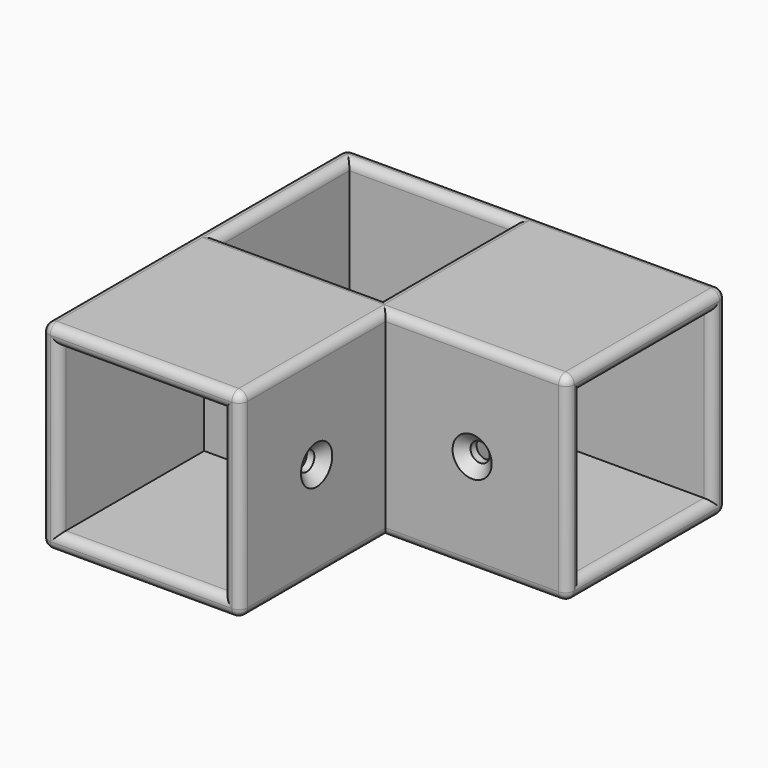
from build123d import *

# Parameters (mm, degrees)
F0_W                  = 34.2
F0_H                  = 34.2
F0_W_2                = 28.2
F0_H_2                = 28.2
F1_DEPTH              = 3
F2_DEPTH              = 31.2
F3_W                  = 34.2
F3_H                  = 34.2
F3_W_2                = 28.2
F3_H_2                = 28.2
F4_DEPTH              = 31.2
F5_W                  = 34.2
F5_H                  = 34.2
F5_W_2                = 28.2
F5_H_2                = 28.2
F6_DEPTH              = 31.2
F7_D                  = 3.3
F7_DEPTH              = 13.5
F7_CSINK_D            = 6.72
F7_CSINK_ANGLE        = 90
F7_TIP                = 0.9914200214
F7_ON_F5_D            = 3.3
F7_ON_F5_DEPTH        = 13.5
F7_ON_F5_CSINK_D      = 6.72
F7_ON_F5_CSINK_ANGLE  = 90
F7_ON_F5_TIP          = 0.9914200214
F7_ON_F3_D            = 3.3
F7_ON_F3_DEPTH        = 13.5
F7_ON_F3_CSINK_D      = 6.72
F7_ON_F3_CSINK_ANGLE  = 90
F7_ON_F3_TIP          = 0.9914200214
F8_R                  = 1.49999
F11_D                 = 3.3
F11_DEPTH             = 13.5
F11_CSINK_D           = 6.72
F11_CSINK_ANGLE       = 90
F11_TIP               = 0.9914200214
F11_ON_F9_D           = 3.3
F11_ON_F9_DEPTH       = 13.5
F11_ON_F9_CSINK_D     = 6.72
F11_ON_F9_CSINK_ANGLE = 90
F11_ON_F9_TIP         = 0.9914200214


# Not quite as in the source:
# - a fillet or chamfer is up to 0.001 mm smaller than in the source, because OpenCascade refuses the exact size


with BuildPart() as f1:
    # F0 (on Top) → F1 (new body)
    with BuildSketch(Plane.XY):
        with Locations((-14.1, 14.1)):
            Rectangle(F0_W, F0_H)
        with Locations((-14.1, 14.1)):
            Rectangle(F0_W_2, F0_H_2, mode=Mode.SUBTRACT)
        with Locations((-14.1, 14.1)):
            Rectangle(F0_W_2, F0_H_2)
    extrude(amount=-F1_DEPTH)

    # F0 (on Top) → F2 (join)
    with BuildSketch(Plane.XY):
        with Locations((-14.1, 14.1)):
            Rectangle(F0_W, F0_H)
        with Locations((-14.1, 14.1)):
            Rectangle(F0_W_2, F0_H_2, mode=Mode.SUBTRACT)
    extrude(amount=F2_DEPTH)

    # F3 (on face) → F4 (join)
    with BuildSketch(Plane.XZ.offset(3)):
        with Locations((-14.1, 14.1)):
            Rectangle(F3_W, F3_H)
        with Locations((-14.1, 14.1)):
            Rectangle(F3_W_2, F3_H_2, mode=Mode.SUBTRACT)
    extrude(amount=F4_DEPTH)

    # F5 (on face) → F6 (join)
    with BuildSketch(Plane.YZ.offset(3)):
        with Locations((14.1, 14.1)):
            Rectangle(F5_W, F5_H)
        with Locations((14.1, 14.1)):
            Rectangle(F5_W_2, F5_H_2, mode=Mode.SUBTRACT)
    extrude(amount=F6_DEPTH)

    # F7
    with Locations(Plane.XY):
        with Locations((-14.1, 14.1)):
            CounterSinkHole(F7_D / 2, F7_CSINK_D / 2, depth=F7_DEPTH, counter_sink_angle=F7_CSINK_ANGLE)
            with Locations((0, 0, -(F7_DEPTH + F7_TIP / 2))):  # 118° drill point
                Cone(0, F7_D / 2, F7_TIP, mode=Mode.SUBTRACT)

    # F7 on F5
    with Locations(Plane.YZ.offset(3)):
        with Locations((14.1, 14.1)):
            CounterSinkHole(F7_ON_F5_D / 2, F7_ON_F5_CSINK_D / 2, depth=F7_ON_F5_DEPTH, counter_sink_angle=F7_ON_F5_CSINK_ANGLE)
            with Locations((0, 0, -(F7_ON_F5_DEPTH + F7_ON_F5_TIP / 2))):  # 118° drill point
                Cone(0, F7_ON_F5_D / 2, F7_ON_F5_TIP, mode=Mode.SUBTRACT)

    # F7 on F3
    with Locations(Plane.XZ.offset(3)):
        with Locations((-14.1, 14.1)):
            CounterSinkHole(F7_ON_F3_D / 2, F7_ON_F3_CSINK_D / 2, depth=F7_ON_F3_DEPTH, counter_sink_angle=F7_ON_F3_CSINK_ANGLE)
            with Locations((0, 0, -(F7_ON_F3_DEPTH + F7_ON_F3_TIP / 2))):  # 118° drill point
                Cone(0, F7_ON_F3_D / 2, F7_ON_F3_TIP, mode=Mode.SUBTRACT)

    # F8 (radius 1.5 in the source; OpenCascade refuses exactly that, so slightly less here)
    f8_edges = [f1.edges().sort_by_distance(p)[0] for p in [
        (-31.2, -1.5, 31.2),
        (1.5, 31.2, 31.2),
        (34.2, 14.1, 31.2),
        (18.6, -3, 31.2),
        (3, -18.6, 31.2),
        (-14.1, -34.2, 31.2),
        (-14.1, 0, 31.2),
        (0, 14.1, 31.2),
        (-28.2, 14.1, 31.2),
        (-14.1, 28.2, 31.2),
        (18.6, -3, -3),
        (3, -18.6, -3),
        (-14.1, -34.2, -3),
        (-31.2, -1.5, -3),
        (1.5, 31.2, -3),
        (34.2, 14.1, -3),
        (3, -34.2, 14.1),
        (0, -34.2, 14.1),
        (-28.2, -34.2, 14.1),
        (-31.2, -34.2, 14.1),
        (-14.1, -34.2, 28.2),
        (-14.1, -34.2, 0),
        (-31.2, 31.2, 14.1),
        (34.2, 31.2, 14.1),
        (34.2, 28.2, 14.1),
        (34.2, 0, 14.1),
        (34.2, -3, 14.1),
        (34.2, 14.1, 0),
        (34.2, 14.1, 28.2),
    ]]
    fillet(f8_edges, radius=F8_R)

    # F11
    with Locations(Plane.XZ.offset(3)):
        with Locations((17.85, 14.1)):
            CounterSinkHole(F11_D / 2, F11_CSINK_D / 2, depth=F11_DEPTH, counter_sink_angle=F11_CSINK_ANGLE)
            with Locations((0, 0, -(F11_DEPTH + F11_TIP / 2))):  # 118° drill point
                Cone(0, F11_D / 2, F11_TIP, mode=Mode.SUBTRACT)

    # F11 on F9
    with Locations(Plane.YZ.offset(3)):
        with Locations((-17.85, 14.1)):
            CounterSinkHole(F11_ON_F9_D / 2, F11_ON_F9_CSINK_D / 2, depth=F11_ON_F9_DEPTH, counter_sink_angle=F11_ON_F9_CSINK_ANGLE)
            with Locations((0, 0, -(F11_ON_F9_DEPTH + F11_ON_F9_TIP / 2))):  # 118° drill point
                Cone(0, F11_ON_F9_D / 2, F11_ON_F9_TIP, mode=Mode.SUBTRACT)


solid = f1.part
